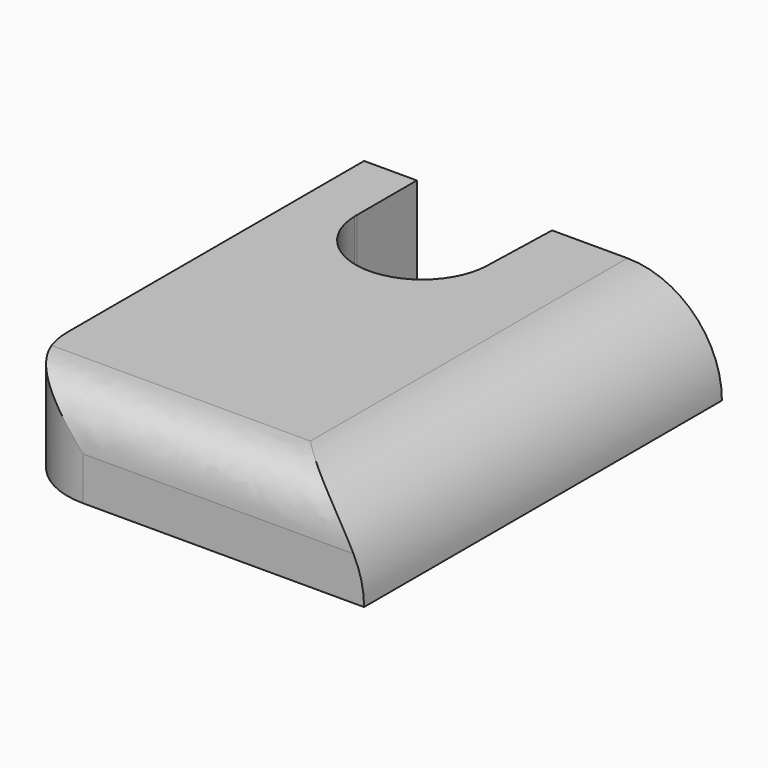
from build123d import *

# Parameters (mm, degrees)
F0_W        = 14
F0_H        = 17.5
F1_DEPTH    = 3.7
F3_DEPTH    = 5.4
F4_R        = 3.69999
F5_R        = 3
F6_T1_DEPTH = 17.30001


# Not quite as in the source:
# - a fillet or chamfer that OpenCascade refuses, or shapes differently, is made with other operations: its cross-section is extruded or revolved along the edge and cut away or added
# - a fillet or chamfer is up to 0.001 mm smaller than in the source, because OpenCascade refuses the exact size


with BuildPart() as f1:
    # F0 (on Top) → F1 (new body)
    with BuildSketch(Plane.XY):
        with Locations((-0.4103374667, 3.4223956802)):
            Rectangle(F0_W, F0_H)
    extrude(amount=F1_DEPTH)

    # F2 (on face) → F3 (cut)
    with BuildSketch(Plane.XY.offset(3.7)):
        with BuildLine():
            Line((-5.3451164257, 9.1307080224), (-5.3451164257, 9.2324278445))
            ThreePointArc((-5.3451164257, 9.2324278445), (-5.3456139214, 9.1815679334), (-5.3451164257, 9.1307080224))
        make_face()
        with BuildLine():
            Line((-5.3451164257, 12.1723956802), (-5.3451164257, 9.2324278445))
            Line((-5.3451164257, 9.2324278445), (-5.3451164257, 9.1307080224))
            ThreePointArc((-5.3451164257, 9.1307080224), (-2.7588797704, 6.5816017765), (-0.1467657558, 9.1041843944))
            Line((-0.1467657558, 9.1041843944), (-0.055406418, 12.1723956802))
            Line((-0.055406418, 12.1723956802), (-5.3451164257, 12.1723956802))
        make_face()
    extrude(amount=-F3_DEPTH, mode=Mode.SUBTRACT)

    # F4 (radius 3.7 in the source; OpenCascade refuses exactly that, so slightly less here)
    f4_edges = [f1.edges().sort_by_distance(p)[0] for p in [
        (6.589663, 3.422396, 3.7),
    ]]
    fillet(f4_edges, radius=F4_R)

    # F5
    f5_edges = [f1.edges().sort_by_distance(p)[0] for p in [
        (-7.410337, -5.327604, 1.85),
    ]]
    fillet(f5_edges, radius=F5_R)

    # F6: fillet of radius 2 on 1 edges, made by hand

    # F6_s2 → F6_t1 (cut)
    with BuildSketch(Plane.YZ.offset(-9.4103374667)):
        with BuildLine():
            add(Edge.make_bspline(
                [(-5.3276043198, 1.7), (-5.3276043198, 3.7), (-3.3276043198, 3.7)],
                knots=[0, 0, 0, 1, 1, 1], degree=2, weights=[1, 1, 1]))
            Line((-3.3276043198, 3.7), (-5.3276043198, 3.7))
            Line((-5.3276043198, 3.7), (-5.3276043198, 1.7))
        make_face()
    extrude(amount=F6_T1_DEPTH, mode=Mode.SUBTRACT)


solid = f1.part
